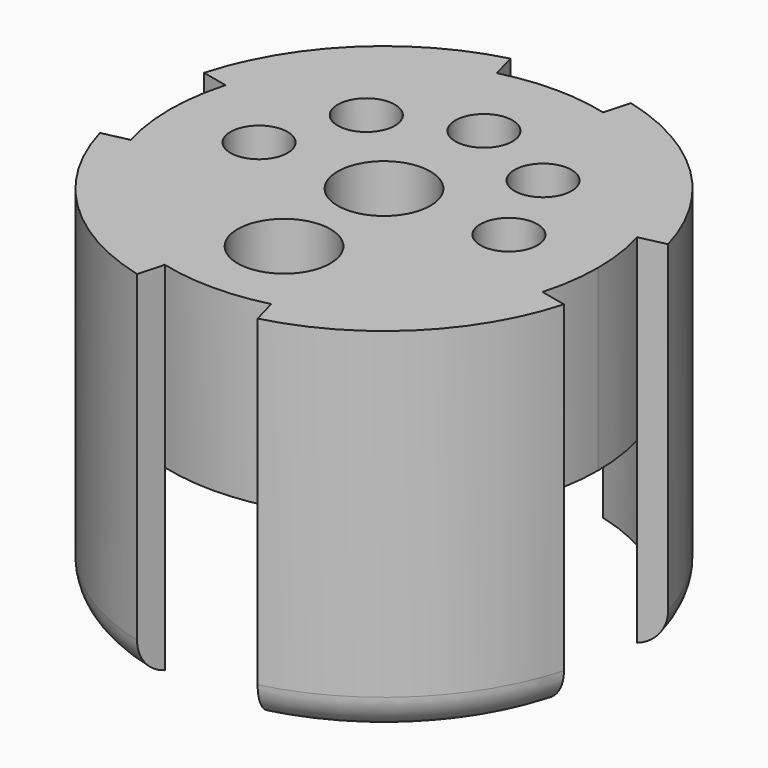
from build123d import *

# Parameters (mm, degrees)
F0_R        = 4.25
F0_R_2      = 2.6
F1_DEPTH    = 10
F0_R_3      = 10.25
F0_R_4      = 1.6
F2_DEPTH    = 10
F3_DEPTH    = 10
F4_DEPTH    = 10
F5_T2_ANGLE = 100.939379093
F5_T4_ANGLE = 100.939379093
F5_T6_ANGLE = 100.939379093
F5_T8_ANGLE = 100.939379093


# Not quite as in the source:
# - a fillet or chamfer that OpenCascade refuses, or shapes differently, is made with other operations: its cross-section is extruded or revolved along the edge and cut away or added


with BuildPart() as f1:
    # F0 (on Top) → F1 (new body)
    with BuildSketch(Plane.XY):
        Circle(F0_R)
        Circle(F0_R_2, mode=Mode.SUBTRACT)
    extrude(amount=F1_DEPTH)

    # F0 (on Top) → F2 (join)
    with BuildSketch(Plane.XY):
        Circle(F0_R_3)
        with Locations((0, -7)):
            Circle(F0_R_2, mode=Mode.SUBTRACT)
        with Locations((-7, 0)):
            Circle(F0_R_4, mode=Mode.SUBTRACT)
        with Locations((-4.95, 4.9494949237)):
            Circle(F0_R_4, mode=Mode.SUBTRACT)
        Circle(F0_R, mode=Mode.SUBTRACT)
        with Locations((4.95, 4.9494949237)):
            Circle(F0_R_4, mode=Mode.SUBTRACT)
        with Locations((7, 0)):
            Circle(F0_R_4, mode=Mode.SUBTRACT)
        with Locations((0, 7)):
            Circle(F0_R_4, mode=Mode.SUBTRACT)
    extrude(amount=F2_DEPTH)

    # F0 (on Top) → F3 (join)
    with BuildSketch(Plane.XY):
        with BuildLine():
            ThreePointArc((11.5318049333, -3.3192581973), (11.8823747458, -1.6760579943), (12, 0))
            ThreePointArc((12, 0), (11.8823747458, 1.6760579943), (11.5318049333, 3.3192581973))
            ThreePointArc((11.5318049333, 3.3192581973), (8.3601945025, 8.6085508583), (2.9803472847, 11.6240066269))
            ThreePointArc((2.9803472847, 11.6240066269), (0, 12), (-2.9803472847, 11.6240066269))
            ThreePointArc((-2.9803472847, 11.6240066269), (-8.3601945025, 8.6085508583), (-11.5318049333, 3.3192581973))
            ThreePointArc((-11.5318049333, 3.3192581973), (-12, 0), (-11.5318049333, -3.3192581973))
            ThreePointArc((-11.5318049333, -3.3192581973), (-8.3601945025, -8.6085508583), (-2.9803472847, -11.6240066269))
            ThreePointArc((-2.9803472847, -11.6240066269), (0, -12), (2.9803472847, -11.6240066269))
            ThreePointArc((2.9803472847, -11.6240066269), (8.3601945025, -8.6085508583), (11.5318049333, -3.3192581973))
        make_face()
        Circle(F0_R_3, mode=Mode.SUBTRACT)
    extrude(amount=F3_DEPTH)

    # F0 (on Top) → F4 (join, symmetric)
    with BuildSketch(Plane.XY):
        with BuildLine():
            ThreePointArc((2.9803472847, 11.6240066269), (8.3601945025, 8.6085508583), (11.5318049333, 3.3192581973))
            Line((11.5318049333, 3.3192581973), (12.9980264072, 3.6470960391))
            ThreePointArc((12.9980264072, 3.6470960391), (9.4466784184, 9.6441830582), (3.3774018659, 13.070698399))
            Line((3.3774018659, 13.070698399), (2.9803472847, 11.6240066269))
        make_face()
        with BuildLine():
            ThreePointArc((-11.5318049333, 3.3192581973), (-8.3601945025, 8.6085508583), (-2.9803472847, 11.6240066269))
            Line((-2.9803472847, 11.6240066269), (-3.3774018659, 13.070698399))
            ThreePointArc((-3.3774018659, 13.070698399), (-9.4466784184, 9.6441830582), (-12.9980264072, 3.6470960391))
            Line((-12.9980264072, 3.6470960391), (-11.5318049333, 3.3192581973))
        make_face()
        with BuildLine():
            Line((-3.3774018659, -13.070698399), (-2.9803472847, -11.6240066269))
            ThreePointArc((-2.9803472847, -11.6240066269), (-8.3601945025, -8.6085508583), (-11.5318049333, -3.3192581973))
            Line((-11.5318049333, -3.3192581973), (-12.9980264072, -3.6470960391))
            ThreePointArc((-12.9980264072, -3.6470960391), (-9.4466784184, -9.6441830582), (-3.3774018659, -13.070698399))
        make_face()
        with BuildLine():
            Line((12.9980264072, -3.6470960391), (11.5318049333, -3.3192581973))
            ThreePointArc((11.5318049333, -3.3192581973), (8.3601945025, -8.6085508583), (2.9803472847, -11.6240066269))
            Line((2.9803472847, -11.6240066269), (3.3774018659, -13.070698399))
            ThreePointArc((3.3774018659, -13.070698399), (9.4466784184, -9.6441830582), (12.9980264072, -3.6470960391))
        make_face()
    extrude(amount=F4_DEPTH, both=True)

    # F5: fillet of radius 2 on 4 edges, made by hand

    # F5_s1 → F5_t2 (revolve, cut)
    with BuildSketch(Plane(origin=(0, 0, 0), x_dir=(0, 0, 1), z_dir=(-0.0850162065, -0.9963795686, 0))):
        with BuildLine():
            ThreePointArc((-10, -12), (-9.2882531983, -13.0811388301), (-8.0635083269, -13.5))
            Line((-8.0635083269, -13.5), (-10, -13.5))
            Line((-10, -13.5), (-10, -12))
        make_face()
    revolve(axis=Axis((0, 0, -10), (0, 0, 1)), revolution_arc=F5_T2_ANGLE, mode=Mode.SUBTRACT)

    # F5_s3 → F5_t4 (revolve, cut)
    with BuildSketch(Plane(origin=(0, 0, 0), x_dir=(0, 0, 1), z_dir=(0.9944074241, -0.1056119072, 0))):
        with BuildLine():
            ThreePointArc((-10, -12), (-9.2882531983, -13.0811388301), (-8.0635083269, -13.5))
            Line((-8.0635083269, -13.5), (-10, -13.5))
            Line((-10, -13.5), (-10, -12))
        make_face()
    revolve(axis=Axis((0, 0, -10), (0, 0, 1)), revolution_arc=F5_T4_ANGLE, mode=Mode.SUBTRACT)

    # F5_s5 → F5_t6 (revolve, cut)
    with BuildSketch(Plane(origin=(0, 0, 0), x_dir=(0, 0, 1), z_dir=(0.0850162065, 0.9963795686, 0))):
        with BuildLine():
            ThreePointArc((-10, -12), (-9.2882531983, -13.0811388301), (-8.0635083269, -13.5))
            Line((-8.0635083269, -13.5), (-10, -13.5))
            Line((-10, -13.5), (-10, -12))
        make_face()
    revolve(axis=Axis((0, 0, -10), (0, 0, 1)), revolution_arc=F5_T6_ANGLE, mode=Mode.SUBTRACT)

    # F5_s7 → F5_t8 (revolve, cut)
    with BuildSketch(Plane(origin=(0, 0, 0), x_dir=(0, 0, 1), z_dir=(-0.9944074241, 0.1056119072, 0))):
        with BuildLine():
            ThreePointArc((-10, -12), (-9.2882531983, -13.0811388301), (-8.0635083269, -13.5))
            Line((-8.0635083269, -13.5), (-10, -13.5))
            Line((-10, -13.5), (-10, -12))
        make_face()
    revolve(axis=Axis((0, 0, -10), (0, 0, 1)), revolution_arc=F5_T8_ANGLE, mode=Mode.SUBTRACT)


solid = f1.part
